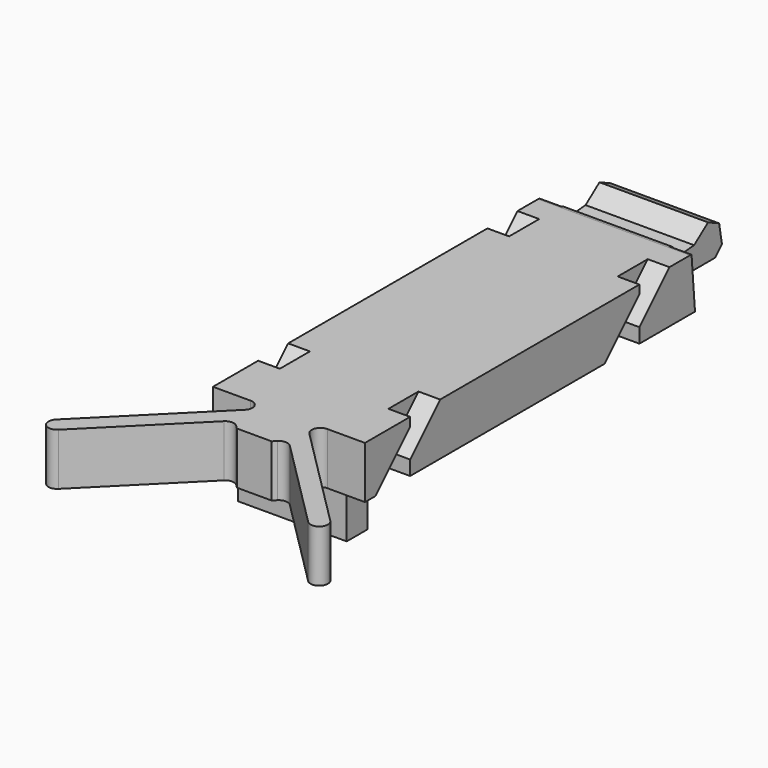
from build123d import *

# Parameters (mm, degrees)
F1_DEPTH  = 8.75
F3_DEPTH  = 2.5
F4_R      = 1
F6_DEPTH  = 6
F8_DEPTH  = 2.5
F9_R      = 1
F11_W     = 9.5
F11_H     = 36
F12_DEPTH = 4
F13_R     = 1


# Not quite as in the source:
# - a feature of the source that left no trace in its solid (it failed there, or was rolled back) is left out
# - a pattern or mirror of a feature is missing from the dataset's text; its kind, count and spacing are read off the source's solid


with BuildPart() as f1:
    # F0 (on Right) → F1 (new body)
    with BuildSketch(Plane.YZ):
        Polygon((3, -5), (3, 0), (47, 0), (49.3, 2.2), (53, 2.2), (54, 3.2), (53.6, 5.45), (52, 6.2), (50, 4.7), (47.5, 4.5), (47, 6), (-0.5, 6), (-0.5, 0), (0, 0), (0, -5), align=None)
    extrude(amount=-F1_DEPTH)

    # F1_copies: F1 across plane


with BuildPart() as f1_1:
    add(f1.part)
    add(f1.part.mirror(Plane(origin=(-8.75, 0, 0), x_dir=(0, 0, -1), z_dir=(-1, 0, 0))))

    # F2 (on face) → F3 (cut)
    with BuildSketch(Plane.YZ):
        Polygon((6, 1.6765981284), (10.3234018716, 6), (6, 6), (6, 5), (1, 0), (-4.5781525858, 0), (-4.5781525858, -7.2408299893), (8, -7.2408299893), (8, 0), (6, 0), align=None)
        Polygon((41, 0), (39, 0), (39, 1.6765981284), (43.3234018716, 6), (39, 6), (39, 5), (34, 0), (28.4218474142, 0), (28.4218474142, -7.2408299893), (41, -7.2408299893), align=None)
        Polygon((74, 0), (72, 0), (72, 1.6765981284), (76.3234018716, 6), (72, 6), (72, 5), (67, 0), (61.4218474142, 0), (61.4218474142, -7.2408299893), (74, -7.2408299893), align=None)
    f3 = extrude(amount=-F3_DEPTH, mode=Mode.SUBTRACT)

    # F3_copies: F3 across plane
    add(f3.mirror(Plane(origin=(-8.75, 0, 0), x_dir=(0, 0, -1), z_dir=(-1, 0, 0))), mode=Mode.SUBTRACT)

    # F4
    f4_edges = [f1_1.edges().sort_by_distance(p)[0] for p in [
        (-8.75, 47, 6),
    ]]
    fillet(f4_edges, radius=F4_R)

    # F5 (on face) → F6 (join, through all)
    with BuildSketch(Plane.XY.offset(6)):
        with BuildLine():
            Line((-6.75, -0.5), (-8.75, -0.5))
            Line((-8.75, -0.5), (-8.75, -5.5))
            Line((-8.75, -5.5), (-6.75, -5.5))
            Line((-6.75, -5.5), (-5.6642135624, -4.4142135624))
            Line((-5.6642135624, -4.4142135624), (5.6286796564, -15.7071067812))
            ThreePointArc((5.6286796564, -15.7071067812), (7.0428932188, -15.7071067812), (7.0428932188, -14.2928932188))
            Line((7.0428932188, -14.2928932188), (-6.75, -0.5))
        make_face()
    f6 = extrude(amount=-F6_DEPTH)

    # F6_copies: F6 across plane
    add(f6.mirror(Plane(origin=(-8.75, 0, 0), x_dir=(0, 0, -1), z_dir=(-1, 0, 0))))

    # F7 (on face) → F8 (cut)
    with BuildSketch(Plane.YZ):
        Polygon((46.5, 7.9169040546), (46.5, 6), (47, 0), (57.128790766, 0), (57.128790766, 7.9169040546), align=None)
    f8 = extrude(amount=-F8_DEPTH, mode=Mode.SUBTRACT)

    # F8_copies: F8 across plane
    add(f8.mirror(Plane(origin=(-8.75, 0, 0), x_dir=(0, 0, -1), z_dir=(-1, 0, 0))), mode=Mode.SUBTRACT)

    # F9
    f9_edges = [f1_1.edges().sort_by_distance(p)[0] for p in [
        (-5.664214, -4.414214, 3),
        (-8.75, 3, 0),
        (-10.75, -0.5, 3),
        (-11.835786, -4.414214, 3),
        (-6.75, -0.5, 3),
    ]]
    fillet(f9_edges, radius=F9_R)

    # F11 (on face) → F12 (cut)
    with BuildSketch(Plane(origin=(0, 0, 0), x_dir=(1, 0, 0), z_dir=(0, 0, -1))):
        with Locations((-8.75, -25)):
            Rectangle(F11_W, F11_H)
    extrude(amount=-F12_DEPTH, mode=Mode.SUBTRACT)

    # F13
    f13_edges = [f1_1.edges().sort_by_distance(p)[0] for p in [
        (-13.5, 7, 2),
        (-4, 7, 2),
        (-13.5, 43, 2),
        (-4, 43, 2),
    ]]
    fillet(f13_edges, radius=F13_R)


solid = f1_1.part
